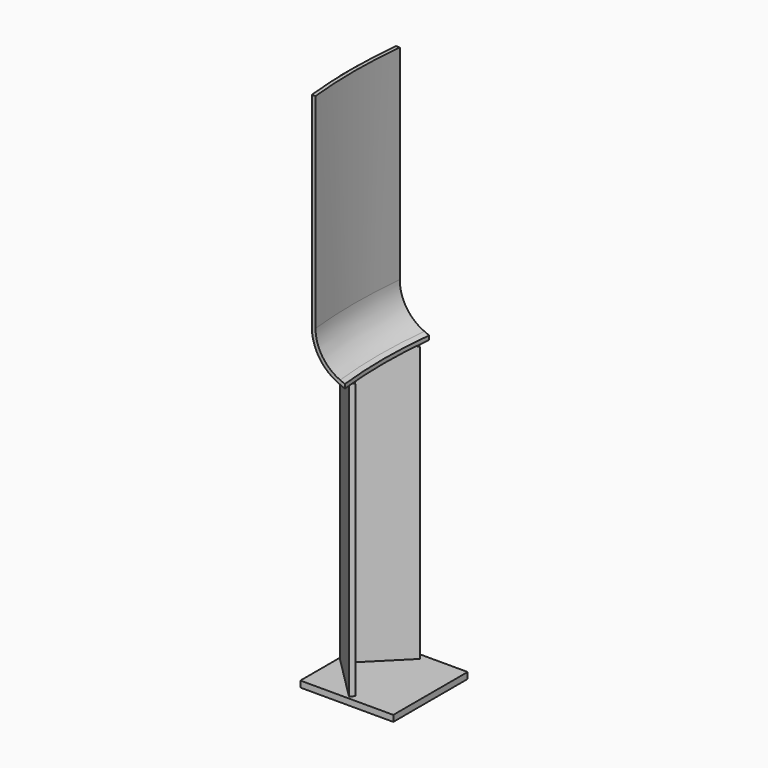
from build123d import *

# Parameters (mm, degrees)
F1_ANGLE_BACK = 15
F1_ANGLE      = 30
F2_W          = 610.7713580132
F2_H          = 748.7817406654
F2_W_2        = 170
F2_H_2        = 405
F3_DEPTH      = 812.0010001
F6_DEPTH      = 845
F5_W          = 150
F5_H          = 150
F7_DEPTH      = 10


with BuildPart() as f1:
    # F0 (on Front) → F1 (revolve)
    with BuildSketch(Plane.XZ, mode=Mode.PRIVATE) as f1_sk:
        with BuildLine():
            ThreePointArc((-759, -228.7132619749), (-762.7450404957, -227.0866981656), (-766.4865952329, -225.4521320796))
            ThreePointArc((-766.4865952329, -225.4521320796), (-795.2454309666, -201.1101420284), (-806, -165))
            Line((-806, -165), (-806, 165))
            Line((-806, 165), (-812, 165))
            Line((-812, 165), (-812, -165))
            ThreePointArc((-812, -165), (-800.2677428727, -204.3928822129), (-768.8944675268, -230.9477804505))
            ThreePointArc((-768.8944675268, -230.9477804505), (-763.9502619939, -233.1057510397), (-759, -235.2497919923))
            Line((-759, -235.2497919923), (-759, -228.713261975))
        make_face()
    revolve(f1_sk.sketch.rotate(Axis((0, 0, -82.5), (0, 0, 1)), -F1_ANGLE_BACK), axis=Axis((0, 0, -82.5), (0, 0, 1)), revolution_arc=F1_ANGLE)

    # F2 (on Right) → F3 (cut, through all)
    with BuildSketch(Plane.YZ):
        Rectangle(F2_W, F2_H)
        with Locations((0, -37.5)):
            Rectangle(F2_W_2, F2_H_2, mode=Mode.SUBTRACT)
    extrude(amount=-F3_DEPTH, mode=Mode.SUBTRACT)


with BuildPart() as f6:
    # F5 (on offset) → F6 (new body)
    with BuildSketch(Plane.XY.offset(-680)):
        Polygon((-759, 70.7106781187), (-829.7106781187, 0), (-759, -70.7106781187), (-753.3431457505, -65.0538238692), (-818.3969696197, 0), (-753.3431457505, 65.0538238692), align=None)
    extrude(amount=F6_DEPTH)

    # F0 (on Front) → F8 (revolve, cut)
    with BuildSketch(Plane.XZ):
        with BuildLine():
            ThreePointArc((-806, -165), (-795.2454309666, -201.1101420284), (-766.4865952329, -225.4521320796))
            ThreePointArc((-766.4865952329, -225.4521320796), (-762.7450404957, -227.0866981656), (-759, -228.7132619749))
            Line((-759, -228.713261975), (-759, 165))
            Line((-759, 165), (-806, 165))
            Line((-806, 165), (-806, -165))
        make_face()
        with BuildLine():
            ThreePointArc((-759, -228.7132619749), (-762.7450404957, -227.0866981656), (-766.4865952329, -225.4521320796))
            ThreePointArc((-766.4865952329, -225.4521320796), (-795.2454309666, -201.1101420284), (-806, -165))
            Line((-806, -165), (-806, 165))
            Line((-806, 165), (-812, 165))
            Line((-812, 165), (-812, -165))
            ThreePointArc((-812, -165), (-800.2677428727, -204.3928822129), (-768.8944675268, -230.9477804505))
            ThreePointArc((-768.8944675268, -230.9477804505), (-763.9502619939, -233.1057510397), (-759, -235.2497919923))
            Line((-759, -235.2497919923), (-759, -228.713261975))
        make_face()
        with BuildLine():
            Line((-759, 165), (-759, -228.713261975))
            ThreePointArc((-759, -228.7132619749), (-734.5550951922, -239.0980108337), (-709.968149662, -249.141839258))
            Line((-709.968149662, -249.141839258), (-709.968149662, -235.2497919923))
            Line((-709.968149662, -235.2497919923), (-709.968149662, 165))
            Line((-709.968149662, 165), (-759, 165))
        make_face()
        with BuildLine():
            ThreePointArc((-709.968149662, -249.141839258), (-734.5550951922, -239.0980108337), (-759, -228.7132619749))
            Line((-759, -228.713261975), (-759, -235.2497919923))
            ThreePointArc((-759, -235.2497919923), (-734.5545744528, -245.5963972216), (-709.968149662, -255.6033341136))
            Line((-709.968149662, -255.6033341136), (-709.968149662, -249.141839258))
        make_face()
    revolve(axis=Axis((0, 0, -272.5), (0, 0, -1)), mode=Mode.SUBTRACT)

    # F0 (on Front) → F9 (revolve, cut)
    with BuildSketch(Plane.XZ):
        Polygon((-842, 140), (-812, 165), (-842, 165), align=None)
    revolve(axis=Axis((0, 0, -272.5), (0, 0, -1)), mode=Mode.SUBTRACT)


with BuildPart() as f7:
    # F5 (on offset) → F7 (new body)
    with BuildSketch(Plane.XY.offset(-680)):
        with Locations((-759, 0)):
            Rectangle(F5_W, F5_H)
        Polygon((-759, -70.7106781187), (-829.7106781187, 0), (-759, 70.7106781187), (-753.3431457505, 65.0538238692), (-818.3969696197, 0), (-753.3431457505, -65.0538238692), align=None, mode=Mode.SUBTRACT)
        Polygon((-759, 70.7106781187), (-829.7106781187, 0), (-759, -70.7106781187), (-753.3431457505, -65.0538238692), (-818.3969696197, 0), (-753.3431457505, 65.0538238692), align=None)
    extrude(amount=-F7_DEPTH)


solid = Compound([f1.part, f6.part, f7.part])
